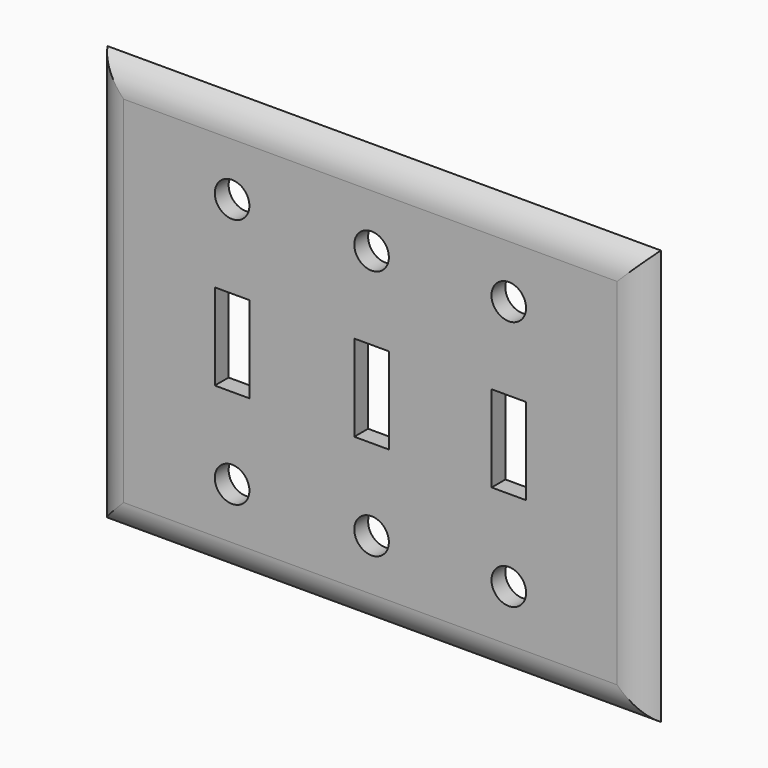
from build123d import *

# Parameters (mm, degrees)
F0_R        = 3.175
F0_W        = 6.35
F0_H        = 15.875
F1_DEPTH    = 3.175
F2_T1_DEPTH = 129.0963065702
F3_T1_DEPTH = 98.1970452562
F4_T1_DEPTH = 98.1970452562
F5_T1_DEPTH = 118.0977839421


# Not quite as in the source:
# - a fillet or chamfer that OpenCascade refuses, or shapes differently, is made with other operations: its cross-section is extruded or revolved along the edge and cut away or added
# - a length typed as a fraction of an inch, garbled in the dataset ("3 / 203.2 mm" for 3/8 in), is restored


with BuildPart() as f1:
    # F0 (on Front) → F1 (new body)
    with BuildSketch(Plane.XZ):
        Polygon((-0.2153298438, 38.1), (-51.0153298438, 38.1), (-51.0153298438, 0), (-51.0153298438, -8.2507394254), (-51.0153298438, -38.1), (50.5846701562, -38.1), (50.5846701562, 7.6242605746), (50.5846701562, 38.1), align=None)
        with Locations((-25.6096087396, -23.1753697127)):
            Circle(F0_R, mode=Mode.SUBTRACT)
        with Locations((-25.6145072252, -0.3132394254)):
            Rectangle(F0_W, F0_H, mode=Mode.SUBTRACT)
        with Locations((0, -23.1753697127)):
            Circle(F0_R, mode=Mode.SUBTRACT)
        with Locations((25.1914858818, -23.1753697127)):
            Circle(F0_R, mode=Mode.SUBTRACT)
        with Locations((-0.0039746718, -0.2589693381)):
            Rectangle(F0_W, F0_H, mode=Mode.SUBTRACT)
        with Locations((25.21736947, -0.2557926551)):
            Rectangle(F0_W, F0_H, mode=Mode.SUBTRACT)
        with Locations((-25.6096087396, 22.8621302873)):
            Circle(F0_R, mode=Mode.SUBTRACT)
        with Locations((0, 22.8621302873)):
            Circle(F0_R, mode=Mode.SUBTRACT)
        with Locations((25.1914858818, 22.8621302873)):
            Circle(F0_R, mode=Mode.SUBTRACT)
    extrude(amount=F1_DEPTH)

    # F2: fillet of radius 6.35 on 1 edges, made by hand

    # F2_s2 → F2_t1 (cut)
    with BuildSketch(Plane.YZ.offset(-64.7634831288)):
        with BuildLine():
            ThreePointArc((0, 38.1), (-2.324261314, 35.775738686), (-3.175, 32.600738686))
            Line((-3.175, 32.600738686), (-3.175, 38.1))
            Line((-3.175, 38.1), (0, 38.1))
        make_face()
    extrude(amount=F2_T1_DEPTH, mode=Mode.SUBTRACT)

    # F3: fillet of radius 6.35 on 1 edges, made by hand

    # F3_s2 → F3_t1 (cut)
    with BuildSketch(Plane.XY.offset(-51.8481532851)):
        with BuildLine():
            ThreePointArc((-51.0153298438, 0), (-48.6910685297, -2.324261314), (-45.5160685297, -3.175))
            Line((-45.5160685297, -3.175), (-51.0153298438, -3.175))
            Line((-51.0153298438, -3.175), (-51.0153298438, 0))
        make_face()
    extrude(amount=F3_T1_DEPTH, mode=Mode.SUBTRACT)

    # F4: fillet of radius 6.35 on 1 edges, made by hand

    # F4_s2 → F4_t1 (cut)
    with BuildSketch(Plane.XY.offset(-51.8481532851)):
        with BuildLine():
            ThreePointArc((50.5846701562, 0), (48.2604088422, -2.324261314), (45.0854088422, -3.175))
            Line((45.0854088422, -3.175), (50.5846701562, -3.175))
            Line((50.5846701562, -3.175), (50.5846701562, 0))
        make_face()
    extrude(amount=F4_T1_DEPTH, mode=Mode.SUBTRACT)

    # F5: fillet of radius 6.35 on 1 edges, made by hand

    # F5_s2 → F5_t1 (cut)
    with BuildSketch(Plane.YZ.offset(-59.2642218148)):
        with BuildLine():
            ThreePointArc((0, -38.1), (-2.324261314, -35.775738686), (-3.175, -32.600738686))
            Line((-3.175, -32.600738686), (-3.175, -38.1))
            Line((-3.175, -38.1), (0, -38.1))
        make_face()
    extrude(amount=F5_T1_DEPTH, mode=Mode.SUBTRACT)


solid = f1.part
